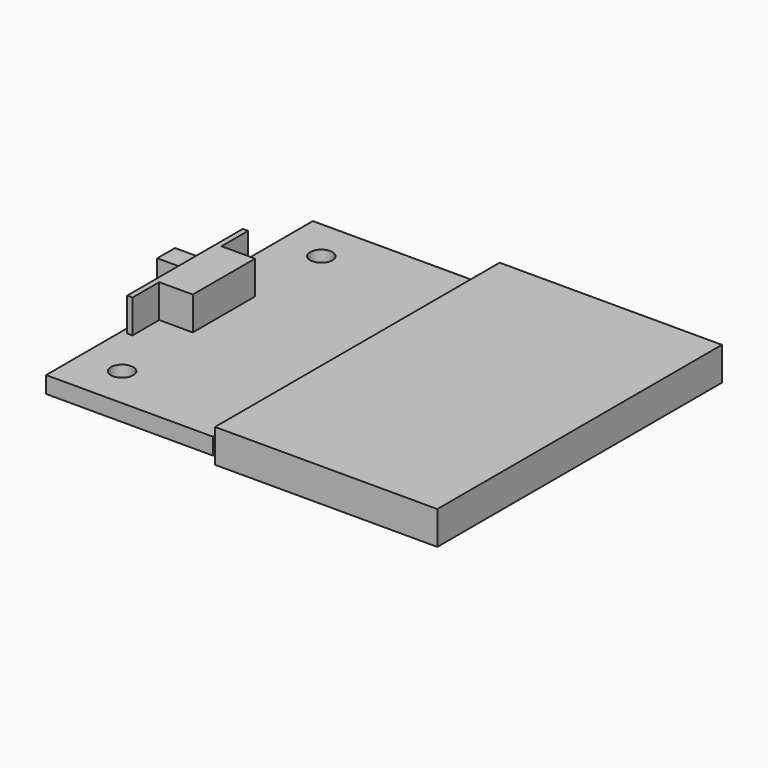
from build123d import *

# Parameters (mm, degrees)
F0_W     = 31.75
F0_H     = 50.8
F1_DEPTH = 4.7625
F2_W     = 23.8125
F2_H     = 47.625
F2_R     = 1.5875
F3_DEPTH = 2.38125
F5_DEPTH = 4.7625
F6_W     = 3.175
F6_H     = 3.175
F7_DEPTH = 3.96875


# Not quite as in the source:
# - a length typed as a fraction of an inch, garbled in the dataset ("3 / 203.2 mm" for 3/8 in), is restored


with BuildPart() as f1:
    # F0 (on Top) → F1 (new body)
    with BuildSketch(Plane.XY):
        with Locations((12.7, 0)):
            Rectangle(F0_W, F0_H)
    extrude(amount=F1_DEPTH)


with BuildPart() as f3:
    # F2 (on Top) → F3 (new body)
    with BuildSketch(Plane.XY):
        with Locations((-16.66875, 0)):
            Rectangle(F2_W, F2_H)
        with Locations((-22.5425, -17.78)):
            Circle(F2_R, mode=Mode.SUBTRACT)
        with Locations((-22.5425, 17.78)):
            Circle(F2_R, mode=Mode.SUBTRACT)
    extrude(amount=F3_DEPTH)


with BuildPart() as f5:
    # F4 (on face) → F5 (new body)
    with BuildSketch(Plane.XY.offset(2.38125)):
        Polygon((-27.01925, 10.31875), (-27.78125, 10.31875), (-27.78125, -10.31875), (-27.01925, -10.31875), (-27.01925, -5.55625), (-22.225, -5.55625), (-22.225, 5.55625), (-27.01925, 5.55625), align=None)
    extrude(amount=F5_DEPTH)

    # F6 (on face) → F7 (join)
    with BuildSketch(Plane(origin=(-27.78125, 0, 0), x_dir=(0, -1, 0), z_dir=(-1, 0, 0))):
        with Locations((-1.5875, 4.7625)):
            Rectangle(F6_W, F6_H)
    extrude(amount=F7_DEPTH)


solid = Compound([f1.part, f3.part, f5.part])
